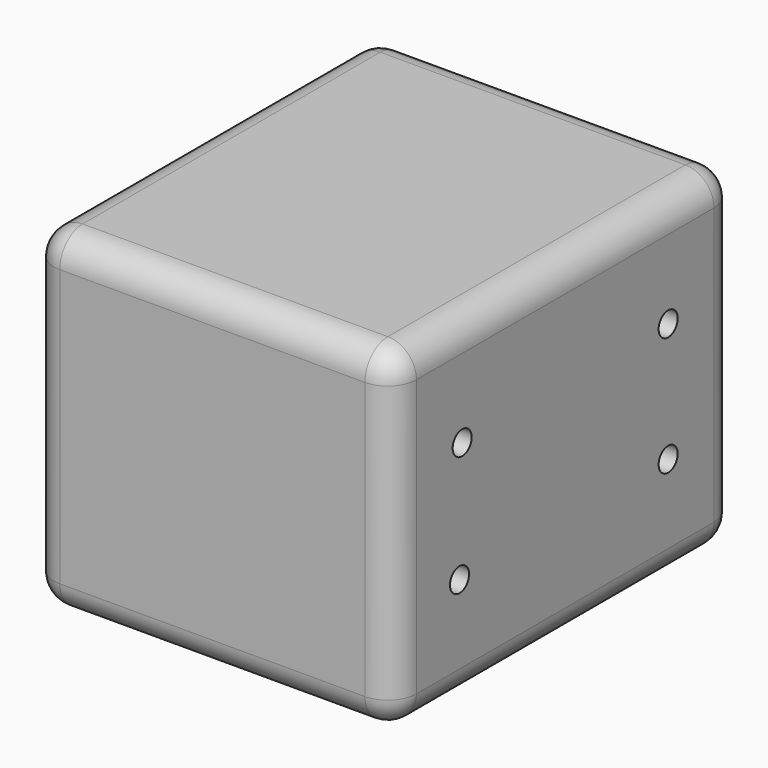
from build123d import *

# Parameters (mm, degrees)
F0_W         = 38
F0_H         = 45
F1_DEPTH     = 35
F2_W         = 13
F2_H         = 25
F2_R         = 1.25
F3_DEPTH     = 16
F4_T1_DEPTH  = 32
F4_T3_DEPTH  = 39
F4_T5_DEPTH  = 29
F4_S9_W      = 3
F4_S9_H      = 3
F4_T10_DEPTH = 3
F4_S15_W     = 3
F4_S15_H     = 3
F4_T16_DEPTH = 3
F4_S21_W     = 3
F4_S21_H     = 3
F4_T22_DEPTH = 3
F4_S27_W     = 3
F4_S27_H     = 3
F4_T28_DEPTH = 3
F4_S33_W     = 3
F4_S33_H     = 3
F4_T34_DEPTH = 3
F4_S39_W     = 3
F4_S39_H     = 3
F4_T40_DEPTH = 3
F4_S45_W     = 3
F4_S45_H     = 3
F4_T46_DEPTH = 3
F4_S51_W     = 3
F4_S51_H     = 3
F4_T52_DEPTH = 3
F5_R         = 1.25
F6_DEPTH     = 7


# Not quite as in the source:
# - a fillet or chamfer that OpenCascade refuses, or shapes differently, is made with other operations: its cross-section is extruded or revolved along the edge and cut away or added


with BuildPart() as f1:
    # F0 (on Top) → F1 (new body)
    with BuildSketch(Plane.XY):
        with Locations((4.8651863657, 11.567664966)):
            Rectangle(F0_W, F0_H)
    extrude(amount=F1_DEPTH)

    # F2 (on face) → F3 (cut)
    with BuildSketch(Plane(origin=(-14.1348136343, 0, 0), x_dir=(0, -1, 0), z_dir=(-1, 0, 0))):
        with Locations((-25.067664966, 17.5)):
            Rectangle(F2_W, F2_H)
        with Locations((1.932335034, 17.5)):
            Rectangle(F2_W, F2_H)
        with Locations((1.932335034, 32.25)):
            Circle(F2_R)
        with Locations((1.932335034, 2.75)):
            Circle(F2_R)
        with Locations((-25.067664966, 32.25)):
            Circle(F2_R)
        with Locations((-25.067664966, 2.75)):
            Circle(F2_R)
    extrude(amount=-F3_DEPTH, mode=Mode.SUBTRACT)

    # F4: fillet of radius 3 on 12 edges, made by hand

    # F4_s2 → F4_t1 (cut)
    with BuildSketch(Plane.YZ.offset(-11.1348136343)):
        with BuildLine():
            ThreePointArc((34.067664966, 3), (33.1889853095, 0.8786796564), (31.067664966, 0))
            Line((31.067664966, 0), (34.067664966, 0))
            Line((34.067664966, 0), (34.067664966, 3))
        make_face()
        with BuildLine():
            ThreePointArc((34.067664966, 32), (33.1889853095, 34.1213203436), (31.067664966, 35))
            Line((31.067664966, 35), (34.067664966, 35))
            Line((34.067664966, 35), (34.067664966, 32))
        make_face()
        with BuildLine():
            ThreePointArc((-7.932335034, 0), (-10.0536553776, 0.8786796564), (-10.932335034, 3))
            Line((-10.932335034, 3), (-10.932335034, 0))
            Line((-10.932335034, 0), (-7.932335034, 0))
        make_face()
        with BuildLine():
            ThreePointArc((-7.932335034, 35), (-10.0536553776, 34.1213203436), (-10.932335034, 32))
            Line((-10.932335034, 32), (-10.932335034, 35))
            Line((-10.932335034, 35), (-7.932335034, 35))
        make_face()
    extrude(amount=F4_T1_DEPTH, mode=Mode.SUBTRACT)

    # F4_s4 → F4_t3 (cut)
    with BuildSketch(Plane.XZ.offset(-31.067664966)):
        with BuildLine():
            ThreePointArc((20.8651863657, 35), (22.9865067092, 34.1213203436), (23.8651863657, 32))
            Line((23.8651863657, 32), (23.8651863657, 35))
            Line((23.8651863657, 35), (20.8651863657, 35))
        make_face()
        with BuildLine():
            ThreePointArc((20.8651863657, 0), (22.9865067092, 0.8786796564), (23.8651863657, 3))
            Line((23.8651863657, 3), (23.8651863657, 0))
            Line((23.8651863657, 0), (20.8651863657, 0))
        make_face()
        with BuildLine():
            ThreePointArc((-14.1348136343, 32), (-13.2561339779, 34.1213203436), (-11.1348136343, 35))
            Line((-11.1348136343, 35), (-14.1348136343, 35))
            Line((-14.1348136343, 35), (-14.1348136343, 32))
        make_face()
        with BuildLine():
            ThreePointArc((-14.1348136343, 3), (-13.2561339779, 0.8786796564), (-11.1348136343, 0))
            Line((-11.1348136343, 0), (-14.1348136343, 0))
            Line((-14.1348136343, 0), (-14.1348136343, 3))
        make_face()
    extrude(amount=F4_T3_DEPTH, mode=Mode.SUBTRACT)

    # F4_s6 → F4_t5 (cut)
    with BuildSketch(Plane.XY.offset(3)):
        with BuildLine():
            ThreePointArc((20.8651863657, 34.067664966), (22.9865067092, 33.1889853095), (23.8651863657, 31.067664966))
            Line((23.8651863657, 31.067664966), (23.8651863657, 34.067664966))
            Line((23.8651863657, 34.067664966), (20.8651863657, 34.067664966))
        make_face()
        with BuildLine():
            ThreePointArc((20.8651863657, -10.932335034), (22.9865067092, -10.0536553776), (23.8651863657, -7.932335034))
            Line((23.8651863657, -7.932335034), (23.8651863657, -10.932335034))
            Line((23.8651863657, -10.932335034), (20.8651863657, -10.932335034))
        make_face()
        with BuildLine():
            ThreePointArc((-14.1348136343, 31.067664966), (-13.2561339779, 33.1889853095), (-11.1348136343, 34.067664966))
            Line((-11.1348136343, 34.067664966), (-14.1348136343, 34.067664966))
            Line((-14.1348136343, 34.067664966), (-14.1348136343, 31.067664966))
        make_face()
        with BuildLine():
            ThreePointArc((-14.1348136343, -7.932335034), (-13.2561339779, -10.0536553776), (-11.1348136343, -10.932335034))
            Line((-11.1348136343, -10.932335034), (-14.1348136343, -10.932335034))
            Line((-14.1348136343, -10.932335034), (-14.1348136343, -7.932335034))
        make_face()
    extrude(amount=F4_T5_DEPTH, mode=Mode.SUBTRACT)


with BuildPart() as f4_tool8:
    # F4_s9 → F4_t10 (new body)
    with BuildSketch(Plane.XZ.offset(-31.067664966)):
        with Locations((22.3651863657, 1.5)):
            Rectangle(F4_S9_W, F4_S9_H)
    extrude(amount=-F4_T10_DEPTH)

    # F4_s11 → F4_t12 (revolve, cut)
    with BuildSketch(Plane(origin=(20.8651863657, 31.067664966, 3), x_dir=(-0.7071067812, 0, 0.7071067812), z_dir=(-0.7071067812, 0, -0.7071067812))):
        with BuildLine():
            ThreePointArc((0, -3), (3, 0), (0, 3))
            Line((0, 3), (0, -3))
        make_face()
    revolve(axis=Axis((20.8651863657, 31.067664966, 3), (0, 1, 0)), mode=Mode.SUBTRACT)


with BuildPart() as f1_1:
    add(f1.part)

    # F4_t7: cut F4_tool8
    add(f4_tool8.part, mode=Mode.SUBTRACT)


with BuildPart() as f4_tool14:
    # F4_s15 → F4_t16 (new body)
    with BuildSketch(Plane.YZ.offset(-11.1348136343)):
        with Locations((32.567664966, 1.5)):
            Rectangle(F4_S15_W, F4_S15_H)
    extrude(amount=-F4_T16_DEPTH)

    # F4_s17 → F4_t18 (revolve, cut)
    with BuildSketch(Plane(origin=(-11.1348136343, 31.067664966, 3), x_dir=(0, -0.7071067812, 0.7071067812), z_dir=(0, -0.7071067812, -0.7071067812))):
        with BuildLine():
            ThreePointArc((0, -3), (3, 0), (0, 3))
            Line((0, 3), (0, -3))
        make_face()
    revolve(axis=Axis((-11.1348136343, 31.067664966, 3), (-1, 0, 0)), mode=Mode.SUBTRACT)


with BuildPart() as f1_2:
    add(f1_1.part)

    # F4_t13: cut F4_tool14
    add(f4_tool14.part, mode=Mode.SUBTRACT)


with BuildPart() as f4_tool20:
    # F4_s21 → F4_t22 (new body)
    with BuildSketch(Plane.XZ.offset(-31.067664966)):
        with Locations((22.3651863657, 33.5)):
            Rectangle(F4_S21_W, F4_S21_H)
    extrude(amount=-F4_T22_DEPTH)

    # F4_s23 → F4_t24 (revolve, cut)
    with BuildSketch(Plane(origin=(20.8651863657, 31.067664966, 32), x_dir=(-0.7071067812, 0, -0.7071067812), z_dir=(0.7071067812, 0, -0.7071067812))):
        with BuildLine():
            ThreePointArc((0, -3), (3, 0), (0, 3))
            Line((0, 3), (0, -3))
        make_face()
    revolve(axis=Axis((20.8651863657, 31.067664966, 32), (0, 1, 0)), mode=Mode.SUBTRACT)


with BuildPart() as f1_3:
    add(f1_2.part)

    # F4_t19: cut F4_tool20
    add(f4_tool20.part, mode=Mode.SUBTRACT)


with BuildPart() as f4_tool26:
    # F4_s27 → F4_t28 (new body)
    with BuildSketch(Plane.YZ.offset(-11.1348136343)):
        with Locations((32.567664966, 33.5)):
            Rectangle(F4_S27_W, F4_S27_H)
    extrude(amount=-F4_T28_DEPTH)

    # F4_s29 → F4_t30 (revolve, cut)
    with BuildSketch(Plane(origin=(-11.1348136343, 31.067664966, 32), x_dir=(0, -0.7071067812, -0.7071067812), z_dir=(0, 0.7071067812, -0.7071067812))):
        with BuildLine():
            ThreePointArc((0, -3), (3, 0), (0, 3))
            Line((0, 3), (0, -3))
        make_face()
    revolve(axis=Axis((-11.1348136343, 31.067664966, 32), (-1, 0, 0)), mode=Mode.SUBTRACT)


with BuildPart() as f1_4:
    add(f1_3.part)

    # F4_t25: cut F4_tool26
    add(f4_tool26.part, mode=Mode.SUBTRACT)


with BuildPart() as f4_tool32:
    # F4_s33 → F4_t34 (new body)
    with BuildSketch(Plane.YZ.offset(-11.1348136343)):
        with Locations((-9.432335034, 1.5)):
            Rectangle(F4_S33_W, F4_S33_H)
    extrude(amount=-F4_T34_DEPTH)

    # F4_s35 → F4_t36 (revolve, cut)
    with BuildSketch(Plane(origin=(-11.1348136343, -7.932335034, 3), x_dir=(0, 0.7071067812, 0.7071067812), z_dir=(0, -0.7071067812, 0.7071067812))):
        with BuildLine():
            ThreePointArc((0, -3), (3, 0), (0, 3))
            Line((0, 3), (0, -3))
        make_face()
    revolve(axis=Axis((-11.1348136343, -7.932335034, 3), (-1, 0, 0)), mode=Mode.SUBTRACT)


with BuildPart() as f1_5:
    add(f1_4.part)

    # F4_t31: cut F4_tool32
    add(f4_tool32.part, mode=Mode.SUBTRACT)


with BuildPart() as f4_tool38:
    # F4_s39 → F4_t40 (new body)
    with BuildSketch(Plane.YZ.offset(20.8651863657)):
        with Locations((-9.432335034, 1.5)):
            Rectangle(F4_S39_W, F4_S39_H)
    extrude(amount=F4_T40_DEPTH)

    # F4_s41 → F4_t42 (revolve, cut)
    with BuildSketch(Plane(origin=(20.8651863657, -7.932335034, 3), x_dir=(0, 0.7071067812, 0.7071067812), z_dir=(0, 0.7071067812, -0.7071067812))):
        with BuildLine():
            ThreePointArc((0, -3), (3, 0), (0, 3))
            Line((0, 3), (0, -3))
        make_face()
    revolve(axis=Axis((20.8651863657, -7.932335034, 3), (1, 0, 0)), mode=Mode.SUBTRACT)


with BuildPart() as f1_6:
    add(f1_5.part)

    # F4_t37: cut F4_tool38
    add(f4_tool38.part, mode=Mode.SUBTRACT)


with BuildPart() as f4_tool44:
    # F4_s45 → F4_t46 (new body)
    with BuildSketch(Plane.YZ.offset(-11.1348136343)):
        with Locations((-9.432335034, 33.5)):
            Rectangle(F4_S45_W, F4_S45_H)
    extrude(amount=-F4_T46_DEPTH)

    # F4_s47 → F4_t48 (revolve, cut)
    with BuildSketch(Plane(origin=(-11.1348136343, -7.932335034, 32), x_dir=(0, 0.7071067812, -0.7071067812), z_dir=(0, 0.7071067812, 0.7071067812))):
        with BuildLine():
            ThreePointArc((0, -3), (3, 0), (0, 3))
            Line((0, 3), (0, -3))
        make_face()
    revolve(axis=Axis((-11.1348136343, -7.932335034, 32), (-1, 0, 0)), mode=Mode.SUBTRACT)


with BuildPart() as f1_7:
    add(f1_6.part)

    # F4_t43: cut F4_tool44
    add(f4_tool44.part, mode=Mode.SUBTRACT)


with BuildPart() as f4_tool50:
    # F4_s51 → F4_t52 (new body)
    with BuildSketch(Plane.YZ.offset(20.8651863657)):
        with Locations((-9.432335034, 33.5)):
            Rectangle(F4_S51_W, F4_S51_H)
    extrude(amount=F4_T52_DEPTH)

    # F4_s53 → F4_t54 (revolve, cut)
    with BuildSketch(Plane(origin=(20.8651863657, -7.932335034, 32), x_dir=(0, 0.7071067812, -0.7071067812), z_dir=(0, -0.7071067812, -0.7071067812))):
        with BuildLine():
            ThreePointArc((0, -3), (3, 0), (0, 3))
            Line((0, 3), (0, -3))
        make_face()
    revolve(axis=Axis((20.8651863657, -7.932335034, 32), (1, 0, 0)), mode=Mode.SUBTRACT)


with BuildPart() as f1_8:
    add(f1_7.part)

    # F4_t49: cut F4_tool50
    add(f4_tool50.part, mode=Mode.SUBTRACT)

    # F5 (on face) → F6 (cut)
    with BuildSketch(Plane.YZ.offset(23.8651863657)):
        with Locations((-1.932335034, 23.75)):
            Circle(F5_R)
        with Locations((-2.2813694086, 11.25)):
            Circle(F5_R)
        with Locations((25.067664966, 23.75)):
            Circle(F5_R)
        with Locations((25.067664966, 11.25)):
            Circle(F5_R)
    extrude(amount=-F6_DEPTH, mode=Mode.SUBTRACT)


solid = f1_8.part
